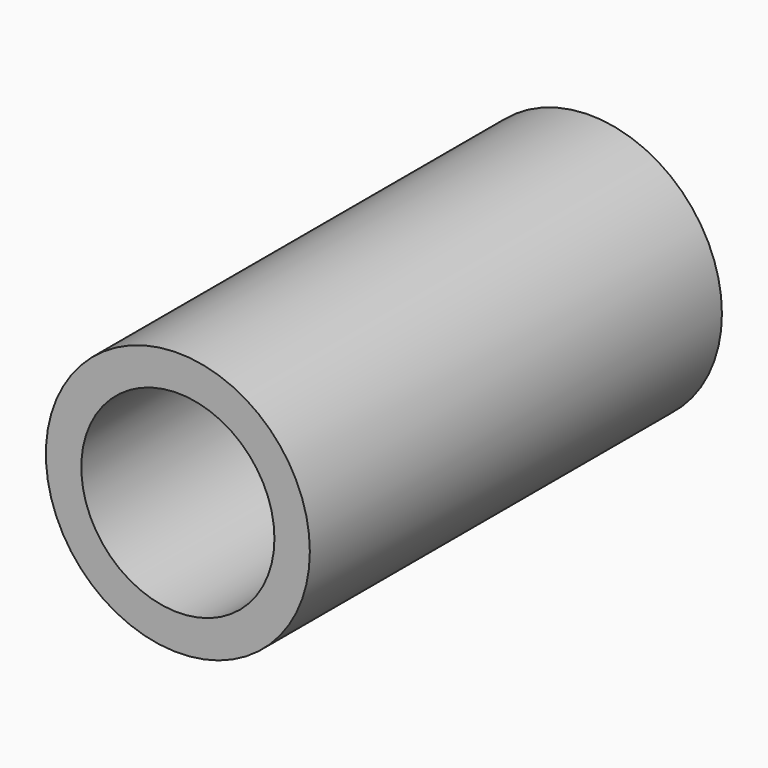
from build123d import *

# Parameters (mm, degrees)
F0_R     = 10.25
F0_R_2   = 7.5
F1_DEPTH = 40
F2_R     = 10.25
F2_R_2   = 7.5
F2_R_3   = 2
F3_DEPTH = 5
F4_R     = 2


with BuildPart() as f1:
    # F0 (on Front) → F1 (new body)
    with BuildSketch(Plane.XZ):
        Circle(F0_R)
        Circle(F0_R_2, mode=Mode.SUBTRACT)
    extrude(amount=-F1_DEPTH)

    # F2 (on face) → F3 (join)
    with BuildSketch(Plane(origin=(0, 40, 0), x_dir=(-1, 0, 0), z_dir=(0, 1, 0))):
        Circle(F2_R)
        Circle(F2_R_2, mode=Mode.SUBTRACT)
        Circle(F2_R_2)
        Circle(F2_R_3, mode=Mode.SUBTRACT)
    extrude(amount=-F3_DEPTH)

    # F4
    f4_edges = [f1.edges().sort_by_distance(p)[0] for p in [
        (2, 35, 0),
    ]]
    fillet(f4_edges, radius=F4_R)


solid = f1.part
